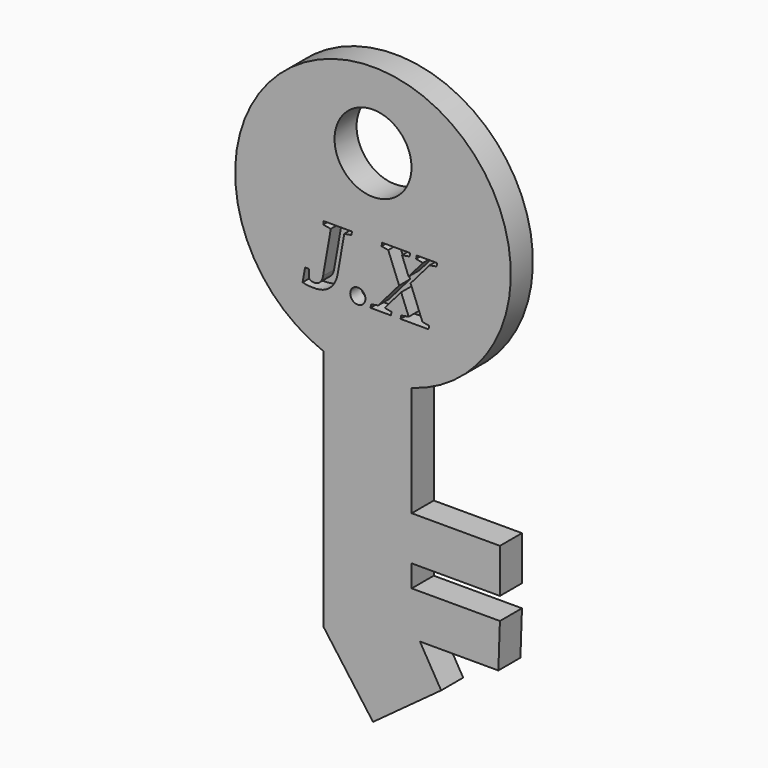
from build123d import *

# Parameters (mm, degrees)
F1_DEPTH     = 3.175
F2_R         = 4.4323962035
F3_DEPTH     = 25.4
F4_TEXT_SIZE = 10.7607054007
F5_DEPTH     = 1.5875


# Not quite as in the source:
# - Text() gives the source's letters only with a copy of the font that has no kerning and outlines rounded to 1/6400 em; it was checked with that copy


with BuildPart() as f1:
    # F0 (on Front) → F1 (new body)
    with BuildSketch(Plane.XZ):
        with BuildLine():
            ThreePointArc((4.4573473037, 13.8301014055), (12.7038579464, 19.5466407799), (15.875, 29.0664946799))
            ThreePointArc((15.875, 29.0664946799), (-8.985711253, 42.1536111796), (-5.7026526963, 14.2511183018))
            ThreePointArc((-5.7026526963, 14.2511183018), (-0.6572748185, 13.2051071362), (4.4573473037, 13.8301014055))
        make_face()
        with BuildLine():
            ThreePointArc((4.4573473037, 13.8301014055), (-0.6572748185, 13.2051071362), (-5.7026526963, 14.2511183018))
            Line((-5.7026526963, 14.2511183018), (-5.7026526963, -13.6888816982))
            Line((-5.7026526963, -13.6888816982), (0, -21.4761056082))
            Line((0, -21.4761056082), (7.84559366, -15.7307082295))
            Line((7.84559366, -15.7307082295), (5.406109198, -11.5666727398))
            Line((5.406109198, -11.5666727398), (14.4363382489, -11.5666727398))
            Line((14.4363382489, -11.5666727398), (14.6173473037, -6.4898985945))
            Line((14.6173473037, -6.4898985945), (4.4573473037, -6.4898985945))
            Line((4.4573473037, -6.4898985945), (4.4573473037, -3.9498985945))
            Line((4.4573473037, -3.9498985945), (14.6173473037, -3.9498985945))
            Line((14.6173473037, -3.9498985945), (14.6173473037, 1.1301014055))
            Line((14.6173473037, 1.1301014055), (4.4573473037, 1.1301014055))
            Line((4.4573473037, 1.1301014055), (4.4573473037, 13.8301014055))
        make_face()
    extrude(amount=F1_DEPTH)

    # F2 (on Front) → F3 (cut)
    with BuildSketch(Plane.XZ):
        with Locations((0, 36.1823962035)):
            Circle(F2_R)
    extrude(amount=F3_DEPTH, mode=Mode.SUBTRACT)

    # F4 (on face) → F5 (cut)
    with BuildSketch(Plane.XZ.offset(3.175)):
        with Locations((-8.0814578919, 20.4122364521)):
            Text('J.X', F4_TEXT_SIZE, font='Tinos', font_style=FontStyle.BOLDITALIC, text_align=(TextAlign.LEFT, TextAlign.BOTTOM))
    extrude(amount=-F5_DEPTH, mode=Mode.SUBTRACT)


solid = f1.part
